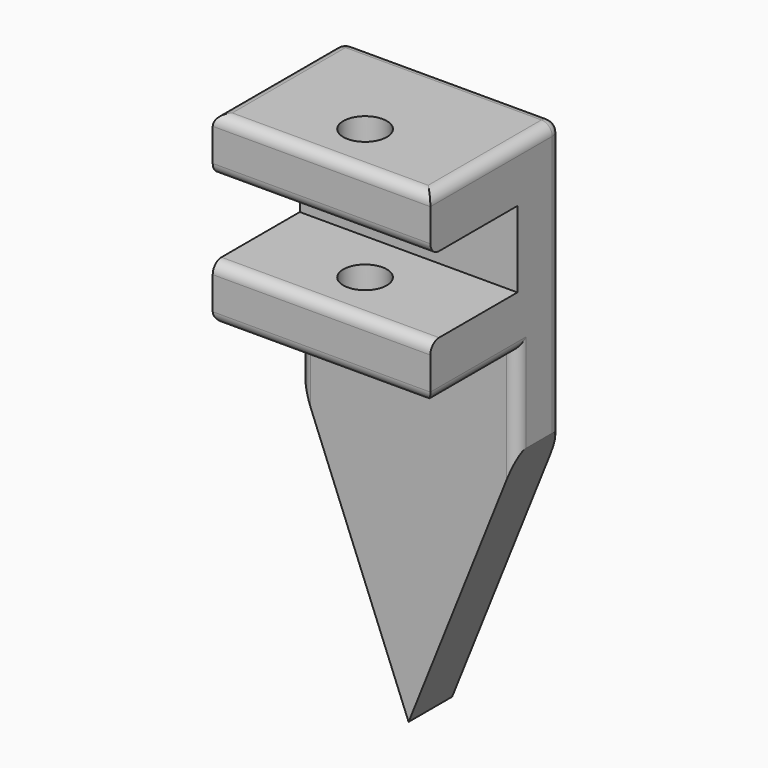
from build123d import *

# Parameters (mm, degrees)
F0_W     = 20
F0_H     = 50
F1_DEPTH = 15
F2_W     = 10
F2_H     = 7
F2_H_2   = 33
F3_DEPTH = 20.001
F5_DEPTH = 15.001
F6_R     = 2
F7_DEPTH = 50.001
F8_R     = 1
F9_R     = 0.99999


# Not quite as in the source:
# - a fillet or chamfer is up to 0.001 mm smaller than in the source, because OpenCascade refuses the exact size


with BuildPart() as f1:
    # F0 (on Front) → F1 (new body)
    with BuildSketch(Plane.XZ):
        Rectangle(F0_W, F0_H)
    extrude(amount=F1_DEPTH)

    # F2 (on face) → F3 (cut, through all)
    with BuildSketch(Plane.YZ.offset(10)):
        with Locations((-10, 16.5)):
            Rectangle(F2_W, F2_H)
        with Locations((-10, -8.5)):
            Rectangle(F2_W, F2_H_2)
    extrude(amount=-F3_DEPTH, mode=Mode.SUBTRACT)

    # F4 (on face) → F5 (cut, through all)
    with BuildSketch(Plane(origin=(0, 0, 0), x_dir=(-1, 0, 0), z_dir=(0, 1, 0))):
        Polygon((0, -25), (-10, 0), (-10, -25), align=None)
        Polygon((10, 0), (0, -25), (10, -25), align=None)
    extrude(amount=-F5_DEPTH, mode=Mode.SUBTRACT)

    # F6 (on face) → F7 (cut, through all)
    with BuildSketch(Plane.XY.offset(25)):
        with Locations((0, -10)):
            Circle(F6_R)
    extrude(amount=-F7_DEPTH, mode=Mode.SUBTRACT)

    # F8
    f8_edges = [f1.edges().sort_by_distance(p)[0] for p in [
        (0, 0, 25),
        (10, -7.5, 25),
        (-10, -7.5, 25),
        (0, -15, 25),
        (10, 0, 12.5),
        (-10, 0, 12.5),
        (-10, -10, 8),
        (10, -10, 8),
        (0, -15, 8),
    ]]
    fillet(f8_edges, radius=F8_R)

    # F9 (radius 1 in the source; OpenCascade refuses exactly that, so slightly less here)
    f9_edges = [f1.edges().sort_by_distance(p)[0] for p in [
        (0, -15, 13),
        (0, -15, 20),
        (-10, -5, 4),
        (10, -5, 4),
    ]]
    fillet(f9_edges, radius=F9_R)


solid = f1.part
